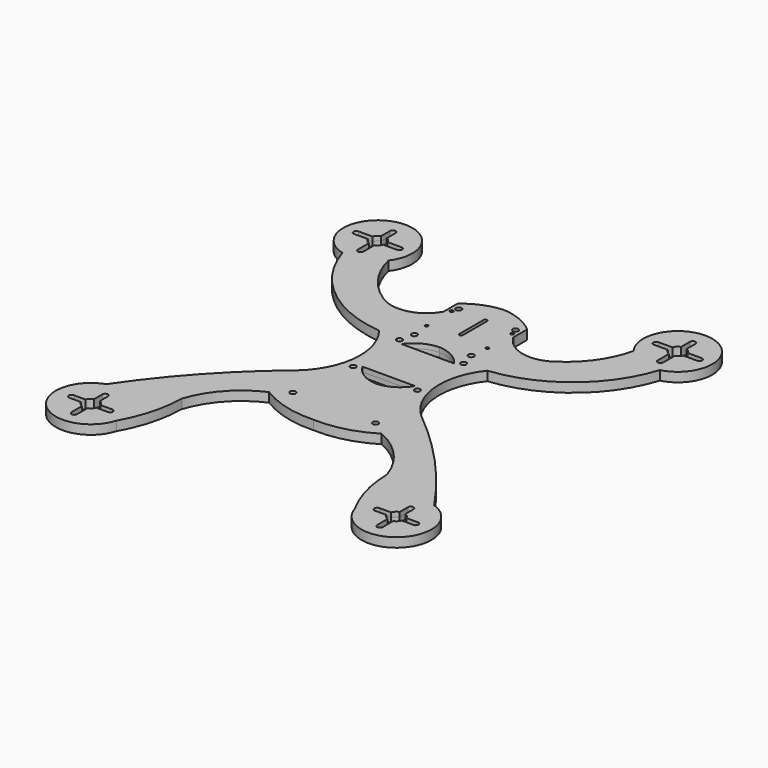
from build123d import *

# Parameters (mm, degrees)
F0_R     = 1.51
F0_R_2   = 1.5
F0_R_3   = 0.8286154485
F1_DEPTH = 2.5


# Not quite as in the source:
# - a feature names something its author has since deleted; it is built from what else it names


with BuildPart() as f1:
    # F0 (on Top) → F1 (new body, symmetric)
    with BuildSketch(Plane.XY):
        with BuildLine():
            Line((-30.1874730734, -52.384633545), (0, -52.384633545))
            Line((0, -52.384633545), (30.1874730734, -52.384633545))
            ThreePointArc((30.1874730734, -52.384633545), (45.5377526982, -63.4637920797), (55.0844569757, -79.8112468001))
            ThreePointArc((55.0844569757, -79.8112468001), (57.4877299486, -96.795391674), (64.006494816, -112.6617902157))
            ThreePointArc((64.006494816, -112.6617902157), (68.9048734281, -93.7156261949), (87.9887831434, -89.3848486541))
            ThreePointArc((87.9887831434, -89.3848486541), (62.7573722568, -57.4704416031), (33.2118480486, -29.5023263287))
            ThreePointArc((33.2118480486, -29.5023263287), (26.7242341229, -24.347436704), (20.0885272052, -19.384633545))
            Line((20.0885272052, -19.384633545), (21.4383106123, 19.6198565499))
            ThreePointArc((21.4383106123, 19.6198565499), (25.2461771825, 19.6733705963), (29.0445808108, 19.9469422451))
            ThreePointArc((29.0445808108, 19.9469422451), (63.9115542942, 34.3327431649), (85.1620762927, 65.494778124))
            ThreePointArc((85.1620762927, 65.494778124), (74.4508574846, 65.9052964442), (65.7591074705, 72.1784308553))
            ThreePointArc((65.7591074705, 72.1784308553), (58.8481462627, 56.5107805649), (46.674050137, 44.4680219955))
            ThreePointArc((46.674050137, 44.4680219955), (45.2140675367, 43.468299654), (43.6672608264, 42.60900753))
            ThreePointArc((43.6672608264, 42.60900753), (31.6040521188, 37.8807075534), (18.7, 36.713118625))
            Line((18.7, 36.713118625), (18.7, 50.3240376711))
            Line((18.7, 50.3240376711), (18.7, 59.615366455))
            ThreePointArc((18.7, 59.615366455), (9.9937787785, 65.0337535356), (0, 67.3319250345))
            ThreePointArc((0, 67.3319250345), (-9.9937787785, 65.0337535356), (-18.7, 59.615366455))
            Line((-18.7, 59.615366455), (-18.7, 50.3240376711))
            Line((-18.7, 50.3240376711), (-18.7, 36.713118625))
            ThreePointArc((-18.7, 36.713118625), (-31.6040521188, 37.8807075534), (-43.6672608264, 42.60900753))
            ThreePointArc((-43.6672608264, 42.60900753), (-45.2140675367, 43.468299654), (-46.674050137, 44.4680219955))
            ThreePointArc((-46.674050137, 44.4680219955), (-58.8481462627, 56.5107805649), (-65.7591074705, 72.1784308553))
            ThreePointArc((-65.7591074705, 72.1784308553), (-74.4508574846, 65.9052964442), (-85.1620762927, 65.494778124))
            ThreePointArc((-85.1620762927, 65.494778124), (-63.9115542942, 34.3327431649), (-29.0445808108, 19.9469422451))
            ThreePointArc((-29.0445808108, 19.9469422451), (-25.2461771825, 19.6733705963), (-21.4383106123, 19.6198565499))
            Line((-21.4383106123, 19.6198565499), (-20.0885272052, -19.384633545))
            ThreePointArc((-20.0885272052, -19.384633545), (-26.7242341229, -24.347436704), (-33.2118480486, -29.5023263287))
            ThreePointArc((-33.2118480486, -29.5023263287), (-62.7573722568, -57.4704416031), (-87.9887831434, -89.3848486541))
            ThreePointArc((-87.9887831434, -89.3848486541), (-71.0247151945, -91.9413319507), (-63.1980110774, -107.2075662893))
            ThreePointArc((-63.1980110774, -107.2075662893), (-63.4012302478, -109.9644759992), (-64.006494816, -112.6617902157))
            ThreePointArc((-64.006494816, -112.6617902157), (-57.4877299486, -96.795391674), (-55.0844569757, -79.8112468001))
            ThreePointArc((-55.0844569757, -79.8112468001), (-45.5377526982, -63.4637920797), (-30.1874730734, -52.384633545))
        make_face()
        with Locations((-22.1585966647, -46.4437194169)):
            Circle(F0_R, mode=Mode.SUBTRACT)
        with Locations((-17.2166451812, -12.1963914914)):
            Circle(F0_R_2, mode=Mode.SUBTRACT)
        with Locations((22.1585966647, -46.4437194169)):
            Circle(F0_R, mode=Mode.SUBTRACT)
        with BuildLine():
            Line((-14.1357257962, -9.8804375157), (0, -9.8804375157))
            Line((0, -9.8804375157), (14.1357257962, -9.8804375157))
            ThreePointArc((14.1357257962, -9.8804375157), (8.1506579233, -15.9532697198), (0, -18.4566881508))
            ThreePointArc((0, -18.4566881508), (-8.1506579233, -15.9532697198), (-14.1357257962, -9.8804375157))
        make_face(mode=Mode.SUBTRACT)
        with Locations((17.2166451812, -12.1963914914)):
            Circle(F0_R_2, mode=Mode.SUBTRACT)
        with BuildLine():
            ThreePointArc((-18.7, 18.5807666779), (-18.7166451812, 18.8036085086), (-18.7, 19.0264503392))
            ThreePointArc((-18.7, 19.0264503392), (-17.1049138701, 20.2994414251), (-15.7166451812, 18.8036085086))
            ThreePointArc((-15.7166451812, 18.8036085086), (-17.1049138701, 17.3077755921), (-18.7, 18.5807666779))
        make_face(mode=Mode.SUBTRACT)
        with Locations((-15.2508411556, 26.3805482537)):
            Circle(F0_R, mode=Mode.SUBTRACT)
        with Locations((-16.3033773307, 35.8986854553)):
            Circle(F0_R_3, mode=Mode.SUBTRACT)
        with BuildLine():
            ThreePointArc((-17.2290705489, 52.7536339848), (-16.3040705489, 53.6786339848), (-15.3790705489, 52.7536339848))
            ThreePointArc((-15.3790705489, 52.7536339848), (-16.3040705489, 51.8286339848), (-17.2290705489, 52.7536339848))
        make_face(mode=Mode.SUBTRACT)
        with Locations((-15.2508411556, 56.1236590147)):
            Circle(F0_R, mode=Mode.SUBTRACT)
        with BuildLine():
            ThreePointArc((-14.1357257962, 16.3518823683), (-7.9488995039, 21.8256144878), (0, 24.0736268461))
            ThreePointArc((0, 24.0736268461), (7.9488995039, 21.8256144878), (14.1357257962, 16.3518823683))
            Line((14.1357257962, 16.3518823683), (0, 16.3518823683))
            Line((0, 16.3518823683), (-14.1357257962, 16.3518823683))
        make_face(mode=Mode.SUBTRACT)
        with BuildLine():
            ThreePointArc((18.7, 18.5807666779), (15.7166451812, 18.8036085086), (18.7, 19.0264503392))
            ThreePointArc((18.7, 19.0264503392), (18.7124780977, 18.9153398197), (18.7166451812, 18.8036085086))
            ThreePointArc((18.7166451812, 18.8036085086), (18.7124780977, 18.6918771974), (18.7, 18.5807666779))
        make_face(mode=Mode.SUBTRACT)
        with Locations((15.2508411556, 26.3805482537)):
            Circle(F0_R, mode=Mode.SUBTRACT)
        with Locations((16.3033773307, 35.8986854553)):
            Circle(F0_R_3, mode=Mode.SUBTRACT)
        with BuildLine():
            ThreePointArc((0.925, 38.6986881495), (0.6540737726, 38.0446143769), (0, 37.7736881495))
            ThreePointArc((0, 37.7736881495), (-0.6540737726, 38.0446143769), (-0.925, 38.6986881495))
            Line((-0.925, 38.6986881495), (-0.925, 54.8593327403))
            ThreePointArc((-0.925, 54.8593327403), (-0.6540737726, 55.5134065129), (0, 55.7843327403))
            ThreePointArc((0, 55.7843327403), (0.6540737726, 55.5134065129), (0.925, 54.8593327403))
            Line((0.925, 54.8593327403), (0.925, 38.6986881495))
        make_face(mode=Mode.SUBTRACT)
        with BuildLine():
            ThreePointArc((15.3790705489, 52.7536339848), (16.3040705489, 53.6786339848), (17.2290705489, 52.7536339848))
            ThreePointArc((17.2290705489, 52.7536339848), (16.3040705489, 51.8286339848), (15.3790705489, 52.7536339848))
        make_face(mode=Mode.SUBTRACT)
        with Locations((15.2508411556, 56.1236590147)):
            Circle(F0_R, mode=Mode.SUBTRACT)
        with BuildLine():
            ThreePointArc((-87.9887831434, -89.3848486541), (-95.0951265719, -120.6995063837), (-64.006494816, -112.6617902157))
            ThreePointArc((-64.006494816, -112.6617902157), (-63.4012302478, -109.9644759992), (-63.1980110774, -107.2075662893))
            ThreePointArc((-63.1980110774, -107.2075662893), (-71.0247151945, -91.9413319507), (-87.9887831434, -89.3848486541))
        make_face()
        with BuildLine():
            ThreePointArc((-80.5, -103.1137172447), (-78.917014434, -104.1245807233), (-77.9061509554, -105.7075662893))
            Line((-77.9061509554, -105.7075662893), (-71.66, -105.7075662893))
            ThreePointArc((-71.66, -105.7075662893), (-70.5993398282, -106.1469061175), (-70.16, -107.2075662893))
            ThreePointArc((-70.16, -107.2075662893), (-70.5993398282, -108.2682264611), (-71.66, -108.7075662893))
            Line((-71.66, -108.7075662893), (-77.9061509554, -108.7075662893))
            ThreePointArc((-77.9061509554, -108.7075662893), (-78.917014434, -110.2905518553), (-80.5, -111.3014153339))
            Line((-80.5, -111.3014153339), (-80.5, -118.2955773668))
            ThreePointArc((-80.5, -118.2955773668), (-82, -119.7955773668), (-83.5, -118.2955773668))
            Line((-83.5, -118.2955773668), (-83.5, -111.3014153339))
            ThreePointArc((-83.5, -111.3014153339), (-85.082985566, -110.2905518553), (-86.0938490446, -108.7075662893))
            Line((-86.0938490446, -108.7075662893), (-92.34, -108.7075662893))
            ThreePointArc((-92.34, -108.7075662893), (-93.84, -107.2075662893), (-92.34, -105.7075662893))
            Line((-92.34, -105.7075662893), (-86.0938490446, -105.7075662893))
            ThreePointArc((-86.0938490446, -105.7075662893), (-85.082985566, -104.1245807233), (-83.5, -103.1137172447))
            Line((-83.5, -103.1137172447), (-83.5, -97.6055773668))
            ThreePointArc((-83.5, -97.6055773668), (-82, -96.1055773668), (-80.5, -97.6055773668))
            Line((-80.5, -97.6055773668), (-80.5, -103.1137172447))
        make_face(mode=Mode.SUBTRACT)
        with BuildLine():
            ThreePointArc((87.9887831434, -89.3848486541), (68.9048734281, -93.7156261949), (64.006494816, -112.6617902157))
            ThreePointArc((64.006494816, -112.6617902157), (84.7569097099, -125.8063360415), (100.8019889226, -107.2075662893))
            ThreePointArc((100.8019889226, -107.2075662893), (97.2662343387, -96.2322814839), (87.9887831434, -89.3848486541))
        make_face()
        with BuildLine():
            Line((83.5, -111.3014153339), (83.5, -118.2955773668))
            ThreePointArc((83.5, -118.2955773668), (82, -119.7955773668), (80.5, -118.2955773668))
            Line((80.5, -118.2955773668), (80.5, -111.3014153339))
            ThreePointArc((80.5, -111.3014153339), (78.917014434, -110.2905518553), (77.9061509554, -108.7075662893))
            Line((77.9061509554, -108.7075662893), (71.66, -108.7075662893))
            ThreePointArc((71.66, -108.7075662893), (70.16, -107.2075662893), (71.66, -105.7075662893))
            Line((71.66, -105.7075662893), (77.9061509554, -105.7075662893))
            ThreePointArc((77.9061509554, -105.7075662893), (78.917014434, -104.1245807233), (80.5, -103.1137172447))
            Line((80.5, -103.1137172447), (80.5, -97.6055773668))
            ThreePointArc((80.5, -97.6055773668), (82, -96.1055773668), (83.5, -97.6055773668))
            Line((83.5, -97.6055773668), (83.5, -103.1137172447))
            ThreePointArc((83.5, -103.1137172447), (85.082985566, -104.1245807233), (86.0938490446, -105.7075662893))
            Line((86.0938490446, -105.7075662893), (92.34, -105.7075662893))
            ThreePointArc((92.34, -105.7075662893), (93.4006601718, -106.1469061175), (93.84, -107.2075662893))
            ThreePointArc((93.84, -107.2075662893), (93.4006601718, -108.2682264611), (92.34, -108.7075662893))
            Line((92.34, -108.7075662893), (86.0938490446, -108.7075662893))
            ThreePointArc((86.0938490446, -108.7075662893), (85.082985566, -110.2905518553), (83.5, -111.3014153339))
        make_face(mode=Mode.SUBTRACT)
        with BuildLine():
            ThreePointArc((-61.9557945169, 83.4250120531), (-91.8151678158, 98.0881017907), (-85.1620762927, 65.494778124))
            ThreePointArc((-85.1620762927, 65.494778124), (-74.4508574846, 65.9052964442), (-65.7591074705, 72.1784308553))
            ThreePointArc((-65.7591074705, 72.1784308553), (-62.932355951, 77.4888774088), (-61.9557945169, 83.4250120531))
        make_face()
        with BuildLine():
            ThreePointArc((-78.9857945169, 87.5188610977), (-77.4028089509, 86.507997619), (-76.3919454723, 84.9250120531))
            Line((-76.3919454723, 84.9250120531), (-68.9257945169, 84.9250120531))
            ThreePointArc((-68.9257945169, 84.9250120531), (-67.8651343451, 84.4856722249), (-67.4257945169, 83.4250120531))
            ThreePointArc((-67.4257945169, 83.4250120531), (-67.8651343451, 82.3643518813), (-68.9257945169, 81.9250120531))
            Line((-68.9257945169, 81.9250120531), (-76.3919454723, 81.9250120531))
            ThreePointArc((-76.3919454723, 81.9250120531), (-77.4028089509, 80.3420264871), (-78.9857945169, 79.3311630085))
            Line((-78.9857945169, 79.3311630085), (-78.9857945169, 71.8650120531))
            ThreePointArc((-78.9857945169, 71.8650120531), (-80.4857945169, 70.3650120531), (-81.9857945169, 71.8650120531))
            Line((-81.9857945169, 71.8650120531), (-81.9857945169, 79.3311630085))
            ThreePointArc((-81.9857945169, 79.3311630085), (-83.5687800828, 80.3420264871), (-84.5796435615, 81.9250120531))
            Line((-84.5796435615, 81.9250120531), (-92.0457945169, 81.9250120531))
            ThreePointArc((-92.0457945169, 81.9250120531), (-93.5457945169, 83.4250120531), (-92.0457945169, 84.9250120531))
            Line((-92.0457945169, 84.9250120531), (-84.5796435615, 84.9250120531))
            ThreePointArc((-84.5796435615, 84.9250120531), (-83.5687800828, 86.507997619), (-81.9857945169, 87.5188610977))
            Line((-81.9857945169, 87.5188610977), (-81.9857945169, 93.4850120531))
            ThreePointArc((-81.9857945169, 93.4850120531), (-80.4857945169, 94.9850120531), (-78.9857945169, 93.4850120531))
            Line((-78.9857945169, 93.4850120531), (-78.9857945169, 87.5188610977))
        make_face(mode=Mode.SUBTRACT)
        with BuildLine():
            ThreePointArc((65.7591074705, 72.1784308553), (74.4508574846, 65.9052964442), (85.1620762927, 65.494778124))
            ThreePointArc((85.1620762927, 65.494778124), (95.1488842545, 72.0956387541), (99.0157945169, 83.4250120531))
            ThreePointArc((99.0157945169, 83.4250120531), (74.5496598725, 100.9784506189), (65.7591074705, 72.1784308553))
        make_face()
        with BuildLine():
            ThreePointArc((81.9857945169, 87.5188610977), (83.5687800828, 86.507997619), (84.5796435615, 84.9250120531))
            Line((84.5796435615, 84.9250120531), (92.0457945169, 84.9250120531))
            ThreePointArc((92.0457945169, 84.9250120531), (93.1064546886, 84.4856722249), (93.5457945169, 83.4250120531))
            ThreePointArc((93.5457945169, 83.4250120531), (93.1064546886, 82.3643518813), (92.0457945169, 81.9250120531))
            Line((92.0457945169, 81.9250120531), (84.5796435615, 81.9250120531))
            ThreePointArc((84.5796435615, 81.9250120531), (83.5687800828, 80.3420264871), (81.9857945169, 79.3311630085))
            Line((81.9857945169, 79.3311630085), (81.9857945169, 71.8650120531))
            ThreePointArc((81.9857945169, 71.8650120531), (80.4857945169, 70.3650120531), (78.9857945169, 71.8650120531))
            Line((78.9857945169, 71.8650120531), (78.9857945169, 79.3311630085))
            ThreePointArc((78.9857945169, 79.3311630085), (77.4028089509, 80.3420264871), (76.3919454723, 81.9250120531))
            Line((76.3919454723, 81.9250120531), (68.9257945169, 81.9250120531))
            ThreePointArc((68.9257945169, 81.9250120531), (67.4257945169, 83.4250120531), (68.9257945169, 84.9250120531))
            Line((68.9257945169, 84.9250120531), (76.3919454723, 84.9250120531))
            ThreePointArc((76.3919454723, 84.9250120531), (77.4028089509, 86.507997619), (78.9857945169, 87.5188610977))
            Line((78.9857945169, 87.5188610977), (78.9857945169, 93.4850120531))
            ThreePointArc((78.9857945169, 93.4850120531), (80.4857945169, 94.9850120531), (81.9857945169, 93.4850120531))
            Line((81.9857945169, 93.4850120531), (81.9857945169, 87.5188610977))
        make_face(mode=Mode.SUBTRACT)
        with BuildLine():
            Line((30.1874730734, -52.384633545), (0, -52.384633545))
            Line((0, -52.384633545), (-30.1874730734, -52.384633545))
            ThreePointArc((-30.1874730734, -52.384633545), (-15.6968009353, -58.6423760096), (0, -60.3004954755))
            ThreePointArc((0, -60.3004954755), (15.6968009353, -58.6423760096), (30.1874730734, -52.384633545))
        make_face()
        with BuildLine():
            ThreePointArc((-29.0445808108, 19.9469422451), (-21.3446813988, -5.6021854639), (-33.2118480486, -29.5023263287))
            ThreePointArc((-33.2118480486, -29.5023263287), (-26.7242341229, -24.347436704), (-20.0885272052, -19.384633545))
            Line((-20.0885272052, -19.384633545), (-21.4383106123, 19.6198565499))
            ThreePointArc((-21.4383106123, 19.6198565499), (-25.2461771825, 19.6733705963), (-29.0445808108, 19.9469422451))
        make_face()
        with BuildLine():
            ThreePointArc((20.0885272052, -19.384633545), (26.7242341229, -24.347436704), (33.2118480486, -29.5023263287))
            ThreePointArc((33.2118480486, -29.5023263287), (21.3446813988, -5.6021854639), (29.0445808108, 19.9469422451))
            ThreePointArc((29.0445808108, 19.9469422451), (25.2461771825, 19.6733705963), (21.4383106123, 19.6198565499))
            Line((21.4383106123, 19.6198565499), (20.0885272052, -19.384633545))
        make_face()
        with BuildLine():
            ThreePointArc((-18.7, 50.3240376711), (-29.6426565817, 41.4796469988), (-43.6672608264, 42.60900753))
            ThreePointArc((-43.6672608264, 42.60900753), (-31.6040521188, 37.8807075534), (-18.7, 36.713118625))
            Line((-18.7, 36.713118625), (-18.7, 50.3240376711))
        make_face()
        with BuildLine():
            ThreePointArc((18.7, 36.713118625), (31.6040521188, 37.8807075534), (43.6672608264, 42.60900753))
            ThreePointArc((43.6672608264, 42.60900753), (29.6426565817, 41.4796469988), (18.7, 50.3240376711))
            Line((18.7, 50.3240376711), (18.7, 36.713118625))
        make_face()
        with BuildLine():
            ThreePointArc((-43.6672608264, 42.60900753), (-45.1885647911, 43.5095480596), (-46.674050137, 44.4680219955))
            ThreePointArc((-46.674050137, 44.4680219955), (-45.2140675367, 43.468299654), (-43.6672608264, 42.60900753))
        make_face()
        with BuildLine():
            Line((-18.7, 18.5807666779), (-18.7, 19.0264503392))
            ThreePointArc((-18.7, 19.0264503392), (-18.7166451812, 18.8036085086), (-18.7, 18.5807666779))
        make_face()
    extrude(amount=F1_DEPTH, both=True)


solid = f1.part
